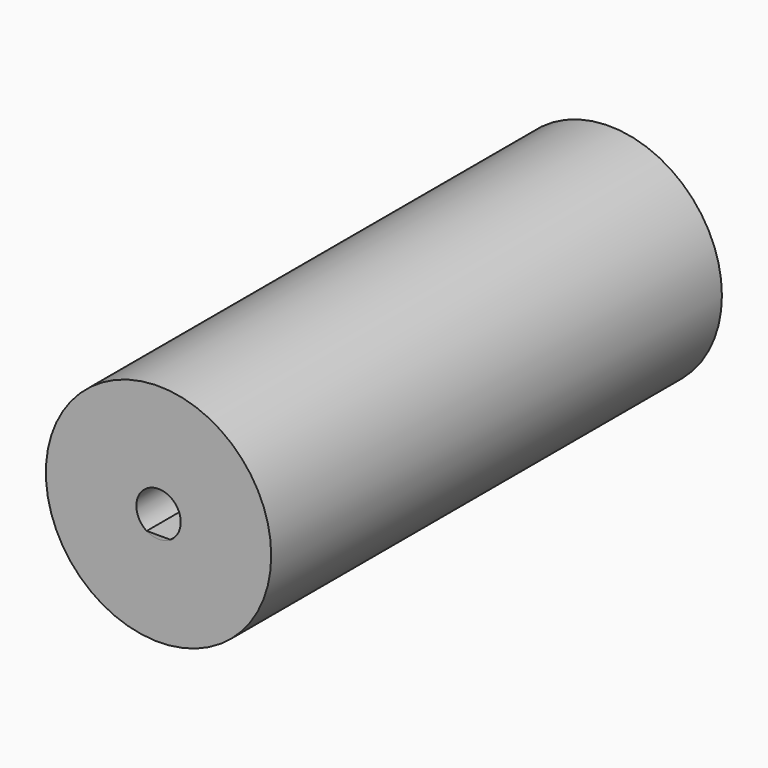
from build123d import *

# Parameters (mm, degrees)
F0_R      = 10.16
F1_DEPTH  = 50.8
F2_R      = 0.25
F3_DEPTH  = 25.4
F5_R      = 12.7
F6_DEPTH  = 31.75
F7_R      = 2.5
F8_DEPTH  = 38.1
F10_DEPTH = 25.4
F11_R     = 1.695
F12_DEPTH = 12.7


with BuildPart() as f1:
    # F0 (on Front) → F1 (new body)
    with BuildSketch(Plane.XZ):
        Circle(F0_R)
    extrude(amount=F1_DEPTH)

    # F2 (on face) → F3 (cut)
    with BuildSketch(Plane.XZ.offset(50.8)):
        Circle(F2_R)
    extrude(amount=-F3_DEPTH, mode=Mode.SUBTRACT)


with BuildPart() as f6:
    # F5 (on Front) → F6 (new body, symmetric)
    with BuildSketch(Plane.XZ):
        Circle(F5_R)
    extrude(amount=F6_DEPTH, both=True)

    # F7 (on face) → F8 (cut)
    with BuildSketch(Plane.XZ.offset(31.75)):
        Circle(F7_R)
    extrude(amount=-F8_DEPTH, mode=Mode.SUBTRACT)

    # F11 (on face) → F12 (cut)
    with BuildSketch(Plane(origin=(0, 31.75, 0), x_dir=(-1, 0, 0), z_dir=(0, 1, 0))):
        Circle(F11_R)
    extrude(amount=-F12_DEPTH, mode=Mode.SUBTRACT)


with BuildPart() as f10:
    # F9 (on face) → F10 (new body)
    with BuildSketch(Plane.XZ.offset(31.75)):
        with BuildLine():
            Line((1.3416786525, -2.1094782278), (0, -2.1094782278))
            Line((0, -2.1094782278), (-1.3416786525, -2.1094782278))
            ThreePointArc((-1.3416786525, -2.1094782278), (0, -2.5), (1.3416786525, -2.1094782278))
        make_face()
    extrude(amount=-F10_DEPTH)


solid = Compound([f6.part, f10.part])
